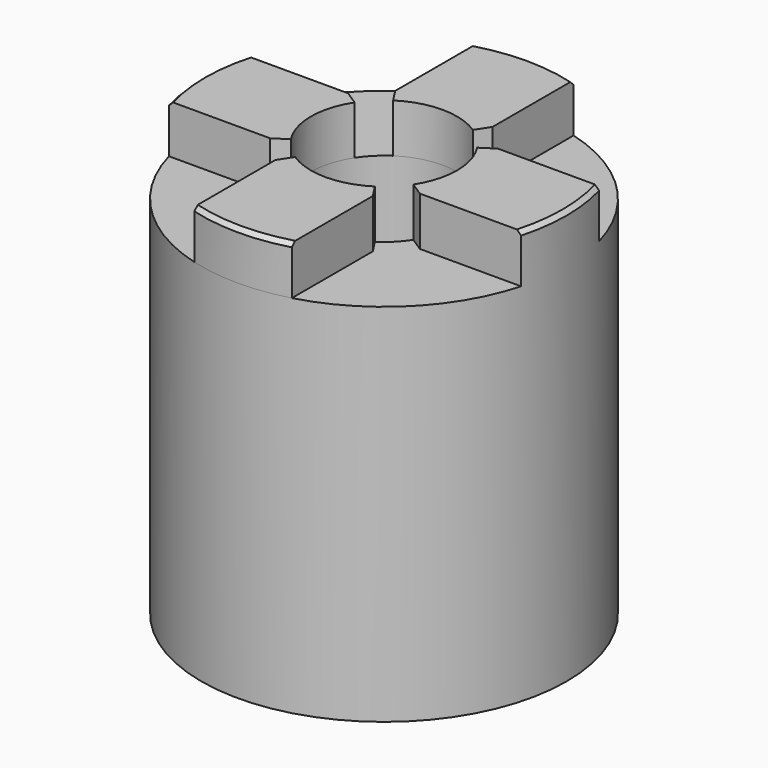
from build123d import *

# Parameters (mm, degrees)
F0_R     = 22.5
F0_R_2   = 9
F1_DEPTH = 45
F3_DEPTH = 6
F4_SIZE  = 0.5


# Not quite as in the source:
# - after a boolean that leaves OpenCascade's solid faulty, fix() repairs it


with BuildPart() as f1:
    # F0 (on Top) → F1 (new body)
    with BuildSketch(Plane.XY):
        Circle(F0_R)
        Circle(F0_R_2, mode=Mode.SUBTRACT)
    extrude(amount=F1_DEPTH)

    # F2 (on face) → F3 (join)
    with BuildSketch(Plane.XY.offset(45)):
        with BuildLine():
            ThreePointArc((-21.6852484422, 6), (-22.5, 0), (-21.6852484422, -6))
            Line((-21.6852484422, -6), (-9.2195444573, -6))
            Line((-9.2195444573, -6), (-7.5432636469, -4.9090909091))
            ThreePointArc((-7.5432636469, -4.9090909091), (-9, 0), (-7.5432636469, 4.9090909091))
            Line((-7.5432636469, 4.9090909091), (-9.2195444573, 6))
            Line((-9.2195444573, 6), (-21.6852484422, 6))
        make_face()
        with BuildLine():
            ThreePointArc((6, 21.6852484422), (0, 22.5), (-6, 21.6852484422))
            Line((-6, 21.6852484422), (-6, 9.2195444573))
            Line((-6, 9.2195444573), (-4.9090909091, 7.5432636469))
            ThreePointArc((-4.9090909091, 7.5432636469), (0, 9), (4.9090909091, 7.5432636469))
            Line((4.9090909091, 7.5432636469), (6, 9.2195444573))
            Line((6, 9.2195444573), (6, 21.6852484422))
        make_face()
        with BuildLine():
            Line((9.2195444573, -6), (21.6852484422, -6))
            ThreePointArc((21.6852484422, -6), (22.2953816961, -3.0275328281), (22.5, 0))
            ThreePointArc((22.5, 0), (22.2953816961, 3.0275328281), (21.6852484422, 6))
            Line((21.6852484422, 6), (9.2195444573, 6))
            Line((9.2195444573, 6), (7.5432636469, 4.9090909091))
            ThreePointArc((7.5432636469, 4.9090909091), (8.6281334257, 2.5603346635), (9, 0))
            ThreePointArc((9, 0), (8.6281334257, -2.5603346635), (7.5432636469, -4.9090909091))
            Line((7.5432636469, -4.9090909091), (9.2195444573, -6))
        make_face()
        with BuildLine():
            Line((-6, -9.2195444573), (-6, -21.6852484422))
            ThreePointArc((-6, -21.6852484422), (0, -22.5), (6, -21.6852484422))
            Line((6, -21.6852484422), (6, -9.2195444573))
            Line((6, -9.2195444573), (4.9090909091, -7.5432636469))
            ThreePointArc((4.9090909091, -7.5432636469), (0, -9), (-4.9090909091, -7.5432636469))
            Line((-4.9090909091, -7.5432636469), (-6, -9.2195444573))
        make_face()
    extrude(amount=F3_DEPTH)

    add(f1.part.fix(), mode=Mode.REPLACE)

    # F4
    f4_edges = [f1.edges().sort_by_distance(p)[0] for p in [
        (-22.5, 0, 51),
        (0, 22.5, 51),
        (22.5, 0, 51),
        (0, -22.5, 51),
    ]]
    chamfer(f4_edges, length=F4_SIZE)


solid = f1.part
